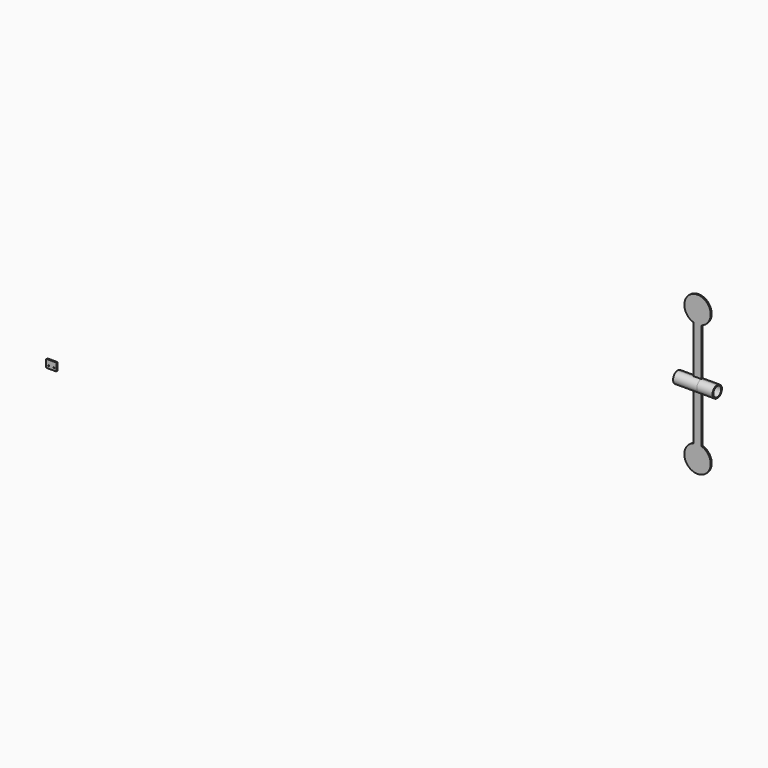
from build123d import *

# Parameters (mm, degrees)
F1_DEPTH = 12.7
F0_R     = 4.7625
F2_R     = 47.12472142
F3_DEPTH = 152.4
F4_DEPTH = 228.6


# Not quite as in the source:
# - a feature names something its author has since deleted; it is built from what else it names


with BuildPart() as f1:
    # F0 (on Front) → F1 (new body)
    with BuildSketch(Plane.XZ):
        with BuildLine():
            Line((-868.383522886, -568.6385392112), (-868.383522886, -111.4385392112))
            ThreePointArc((-868.383522886, -111.4385392112), (-906.483522886, 136.7117393687), (-944.583522886, -111.4385392112))
            Line((-944.583522886, -111.4385392112), (-944.583522886, -568.6385392112))
            Line((-944.583522886, -568.6385392112), (-868.383522886, -568.6385392112))
        make_face()
    extrude(amount=F1_DEPTH)


with BuildPart() as f1b:
    # F0 (on Front) → F1, piece 2 (new body)
    with BuildSketch(Plane.XZ):
        with BuildLine():
            Line((-944.583522886, -681.9379820513), (-944.583522886, -1139.1379820513))
            ThreePointArc((-944.583522886, -1139.1379820513), (-906.483522886, -1387.2882606313), (-868.383522886, -1139.1379820513))
            Line((-868.383522886, -1139.1379820513), (-868.383522886, -681.9379820513))
            Line((-868.383522886, -681.9379820513), (-944.583522886, -681.9379820513))
        make_face()
    extrude(amount=F1_DEPTH)


with BuildPart() as f1c:
    # F0 (on Front) → F1, piece 3 (new body)
    with BuildSketch(Plane.XZ):
        with BuildLine():
            Line((-7101.1272773743, -2454.1268432617), (-7190.0272773743, -2454.1268432617))
            ThreePointArc((-7190.0272773743, -2454.1268432617), (-7194.5174054348, -2455.9867152012), (-7196.3772773743, -2460.4768432617))
            Line((-7196.3772773743, -2460.4768432617), (-7196.3772773743, -2523.9768432617))
            ThreePointArc((-7196.3772773743, -2523.9768432617), (-7194.5174054348, -2528.4669713223), (-7190.0272773743, -2530.3268432617))
            Line((-7190.0272773743, -2530.3268432617), (-7101.1272773743, -2530.3268432617))
            ThreePointArc((-7101.1272773743, -2530.3268432617), (-7096.6371493137, -2528.4669713223), (-7094.7772773743, -2523.9768432617))
            Line((-7094.7772773743, -2523.9768432617), (-7094.7772773743, -2460.4768432617))
            ThreePointArc((-7094.7772773743, -2460.4768432617), (-7096.6371493137, -2455.9867152012), (-7101.1272773743, -2454.1268432617))
        make_face()
        with Locations((-7170.9772773743, -2504.9268432617)):
            Circle(F0_R, mode=Mode.SUBTRACT)
        with Locations((-7120.1772773743, -2504.9268432617)):
            Circle(F0_R, mode=Mode.SUBTRACT)
    extrude(amount=F1_DEPTH)


with BuildPart() as f3:
    # F2 (on face) → F3 (new body)
    with BuildSketch(Plane.YZ.offset(-868.383522886)):
        with BuildLine():
            ThreePointArc((-12.7000001128, -568.638610381), (-52.8789346424, -665.3139022013), (43.8599243822, -625.2882606313))
            ThreePointArc((43.8599243822, -625.2882606313), (27.2993405667, -585.2626190613), (-12.7000001128, -568.638610381))
        make_face()
        with Locations((-12.7897970378, -625.2882606313)):
            Circle(F2_R, mode=Mode.SUBTRACT)
    extrude(amount=F3_DEPTH)


with BuildPart() as f4:
    # F4 (new): a face of the model
    f4_faces = [f3.part.faces().sort_by_distance(p)[0] for p in [
        (-868.383522886, -67.8372223712, -625.2882606313),
    ]]
    extrude(f4_faces, amount=F4_DEPTH)


solid = Compound([f1.part, f1b.part, f1c.part, f3.part, f4.part])
